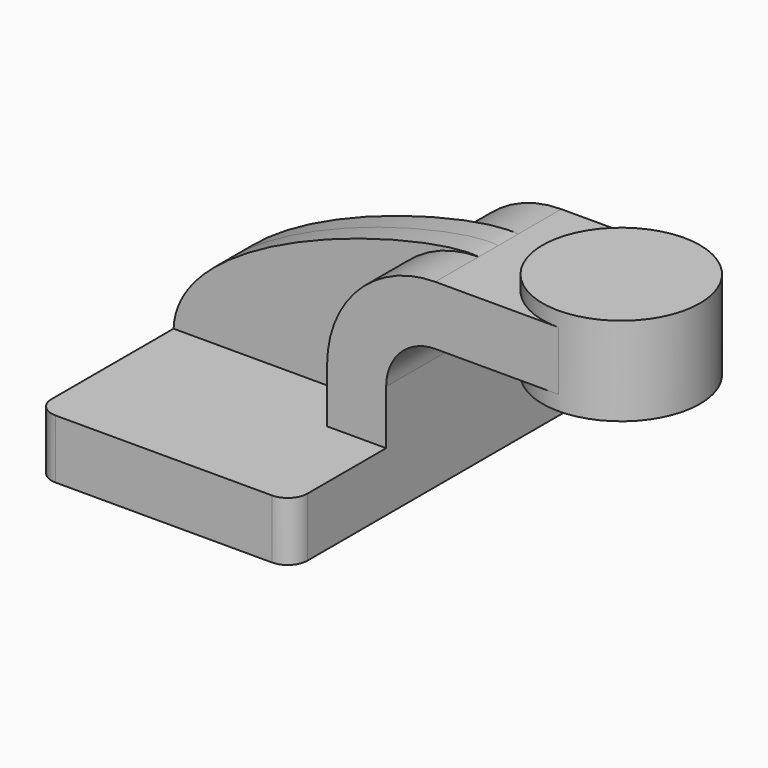
from build123d import *

# Parameters (mm, degrees)
F1_DEPTH = 63.5
F2_DEPTH = 25.4
F3_DEPTH = 7.9375
F5_R     = 6.35


# Not quite as in the source:
# - ends of sketch curves that miss each other by under 0.0002 mm in the source are joined
# - a feature names something its author has since deleted; it is built from what else it names


with BuildPart() as f1:
    # F0 (on Front) → F1 (new body, symmetric)
    with BuildSketch(Plane.XZ):
        Polygon((-41.275, 9.525), (-41.275, -9.525), (41.275, -9.525), (41.275, 9.525), (22.225, 9.525), align=None)
    extrude(amount=F1_DEPTH, both=True)

    # F0 (on Front) → F2 (join, symmetric)
    with BuildSketch(Plane.XZ):
        with BuildLine():
            Line((22.225, 9.525), (41.275, 9.525))
            Line((41.275, 9.525), (41.275, 27.0002))
            ThreePointArc((41.275, 27.0002), (45.9246798487, 38.2255201513), (57.15, 42.8752))
            Line((57.15, 42.8752), (71.4156685244, 42.8752))
            Line((71.4156685244, 42.8752), (71.4156685244, 61.9252))
            Line((71.4156685244, 61.9252), (57.15, 61.9252))
            ThreePointArc((57.15, 61.9252), (32.4542956671, 51.6959043329), (22.225, 27.0002))
            Line((22.225, 27.0002), (22.225, 9.525))
        make_face()
        Polygon((96.8156695652, 61.9252), (71.4156685244, 61.9252), (71.4156685244, 42.8752), (96.8156754971, 42.8752), align=None)
    extrude(amount=F2_DEPTH, both=True)

    # F0 (on Front) → F3 (join, symmetric)
    with BuildSketch(Plane.XZ):
        with BuildLine():
            add(Edge.make_bspline(
                [(-41.275, 9.525), (-40.0072485209, 41.9578626752), (41.6273023615, 64.213483679), (57.15, 61.9252)],
                knots=[0, 0, 0, 0, 111.5045361635, 111.5045361635, 111.5045361635, 111.5045361635], degree=3))
            Line((-41.275, 9.525), (22.225, 9.525))
            Line((22.225, 9.525), (22.225, 27.0002))
            ThreePointArc((22.225, 27.0002), (32.4542956671, 51.6959043329), (57.15, 61.9252))
        make_face()
    extrude(amount=F3_DEPTH, both=True)

    # F0 (on Front) → F4 (revolve)
    with BuildSketch(Plane.XZ):
        Polygon((96.8156685244, 66.675), (96.8156685244, 61.9252), (96.8156685244, 42.8752), (96.8156685244, 38.1), (122.2156685244, 38.1), (122.2156685244, 66.675), align=None)
    revolve(axis=Axis((96.8156685244, 0, 52.3875), (0, 0, 1)))

    # F5
    f5_edges = [f1.edges().sort_by_distance(p)[0] for p in [
        (-41.275, -63.5, 0),
        (-41.275, 63.5, 0),
        (41.275, 63.5, 0),
        (41.275, -63.5, 0),
    ]]
    fillet(f5_edges, radius=F5_R)


solid = f1.part
